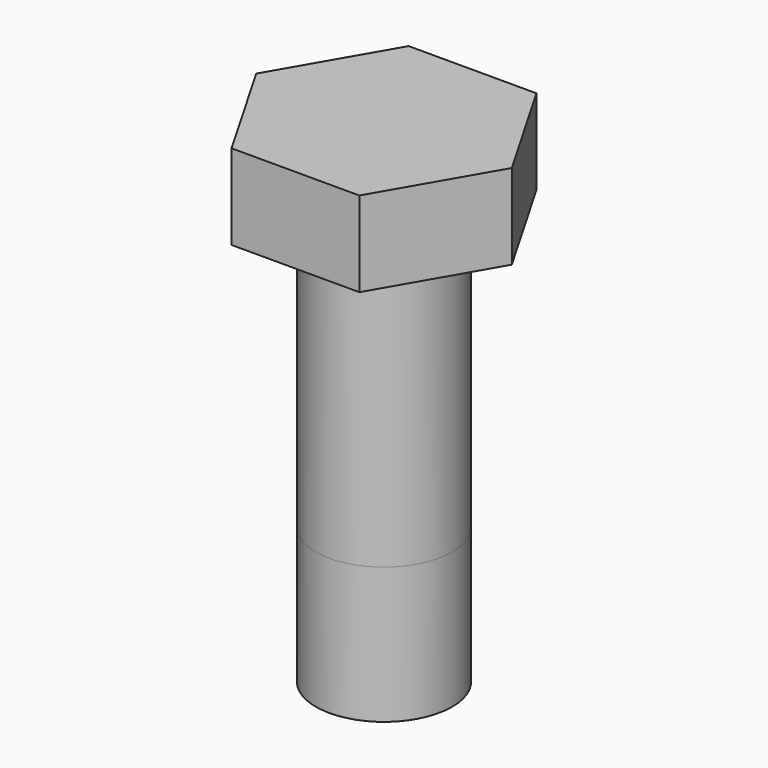
from build123d import *

# Parameters (mm, degrees)
F0_R          = 12.7
F1_DEPTH      = 25.4
F1_DEPTH_BACK = 50.8
F3_DEPTH      = 15.875


# Not quite as in the source:
# - a feature names something its author has since deleted; it is built from what else it names


with BuildPart() as f1:
    # F0 (on Top) → F1 (new body, two sides)
    with BuildSketch(Plane.XY) as f1_sk:
        Circle(F0_R)
    extrude(amount=-F1_DEPTH)
    extrude(f1_sk.sketch, amount=F1_DEPTH_BACK)

    # F2 (on face) → F3 (join)
    with BuildSketch(Plane.XY.offset(50.8)):
        Polygon((11.9150661804, 20.6375), (-11.9150661804, 20.6375), (-23.8301323608, 0), (-11.9150661804, -20.6375), (11.9150661804, -20.6375), (23.8301323608, 0), align=None)
    extrude(amount=F3_DEPTH)


solid = f1.part
